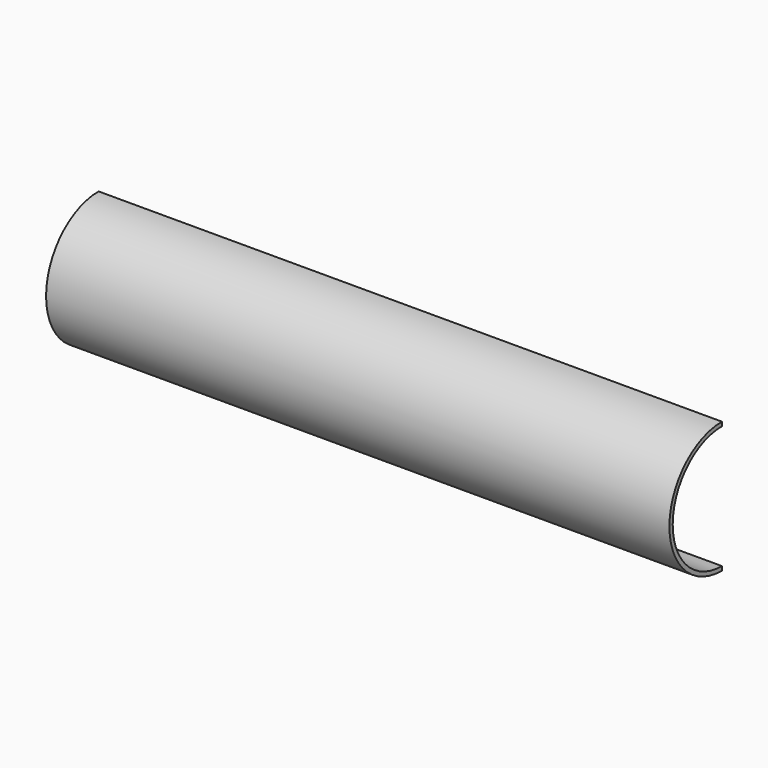
from build123d import *

# Parameters (mm, degrees)
F0_R      = 50.8
F0_R_2    = 47.625
F1_DEPTH  = 482.6
F4_DEPTH  = 508
F5_W      = 55.5464364588
F5_H      = 92.0769795775
F6_DEPTH  = 508
F7_W      = 106.5891161561
F7_H      = 48.0401627719
F8_DEPTH  = 101.6
F9_W      = 58.4661662579
F9_H      = 32.7058173716
F10_DEPTH = 82.55


# Not quite as in the source:
# - the program builds the solid bodies; features that only make, move or delete a surface that nothing else refers to are left out


with BuildPart() as f1:
    # F0 (on Right) → F1 (new body)
    with BuildSketch(Plane.YZ):
        Circle(F0_R)
        Circle(F0_R_2, mode=Mode.SUBTRACT)
    extrude(amount=F1_DEPTH)

    # F3 (on Right) → F4 (cut)
    with BuildSketch(Plane.YZ):
        Polygon((0, 91.0463854671), (0, 0), (0, -77.0941823721), (61.9923658669, -77.0941823721), (61.9923658669, 91.0463854671), align=None)
    extrude(amount=F4_DEPTH, mode=Mode.SUBTRACT)

    # F5 (on Right) → F6 (cut)
    with BuildSketch(Plane.YZ):
        with Locations((27.7732182294, 46.0384897888)):
            Rectangle(F5_W, F5_H)
    extrude(amount=F6_DEPTH, mode=Mode.SUBTRACT)

    # F7 (on Top) → F8 (cut)
    with BuildSketch(Plane.XY):
        with Locations((53.2945580781, 24.020081386)):
            Rectangle(F7_W, F7_H)
    extrude(amount=F8_DEPTH, mode=Mode.SUBTRACT)

    # F9 (on Top) → F10 (cut)
    with BuildSketch(Plane.XY):
        with Locations((77.5640532374, 16.3529086858)):
            Rectangle(F9_W, F9_H)
    extrude(amount=F10_DEPTH, mode=Mode.SUBTRACT)


solid = f1.part
